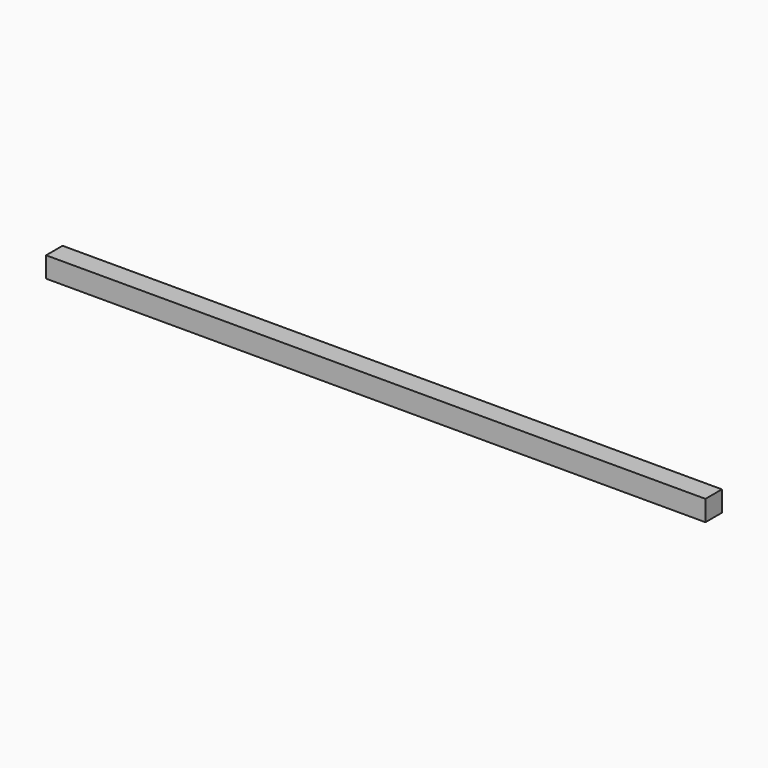
from build123d import *

# Parameters (mm, degrees)
F0_W     = 101.6
F0_H     = 3.175
F1_DEPTH = 3.175


# Not quite as in the source:
# - a length typed as a fraction of an inch, garbled in the dataset ("3 / 203.2 mm" for 3/8 in), is restored


with BuildPart() as f1:
    # F0 (on Front) → F1 (new body)
    with BuildSketch(Plane.XZ):
        Rectangle(F0_W, F0_H)
    extrude(amount=F1_DEPTH)


solid = f1.part
